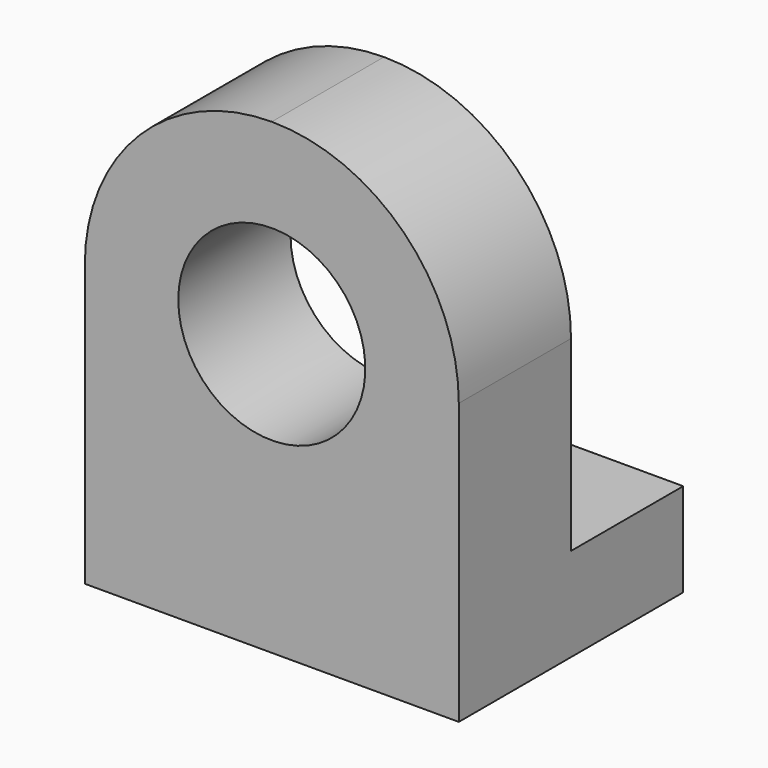
from build123d import *

# Parameters (mm, degrees)
F0_W     = 50.8
F0_H     = 38.1
F1_DEPTH = 6.35
F2_W     = 12.7
F2_H     = 12.7
F3_DEPTH = 12.701
F4_W     = 50.8
F4_H     = 19.05
F5_DEPTH = 50.8
F7_DEPTH = 19.051
F6_R     = 12.7
F8_DEPTH = 19.051


# Not quite as in the source:
# - a feature names something its author has since deleted; it is built from what else it names


with BuildPart() as f1:
    # F0 (on Top) → F1 (new body, symmetric)
    with BuildSketch(Plane.XY):
        Rectangle(F0_W, F0_H)
    extrude(amount=F1_DEPTH, both=True)

    # F2 (on face) → F3 (cut, through all)
    with BuildSketch(Plane.XY.offset(6.35)):
        with Locations((-19.05, 12.7)):
            Rectangle(F2_W, F2_H)
    extrude(amount=-F3_DEPTH, mode=Mode.SUBTRACT)

    # F4 (on face) → F5 (join)
    with BuildSketch(Plane.XY.offset(6.35)):
        with Locations((0, -9.525)):
            Rectangle(F4_W, F4_H)
    extrude(amount=F5_DEPTH)

    # F6 (on face) → F7 (cut, through all)
    with BuildSketch(Plane(origin=(0, 0, 0), x_dir=(-1, 0, 0), z_dir=(0, 1, 0))):
        with BuildLine():
            ThreePointArc((-25.4, 31.75), (-17.9605122618, 49.7105122225), (-5.57e-08, 57.15))
            Line((-5.57e-08, 57.15), (-25.4, 57.15))
            Line((-25.4, 57.15), (-25.4, 31.75))
        make_face()
        with BuildLine():
            ThreePointArc((-5.57e-08, 57.15), (17.9605122225, 49.7105122618), (25.4, 31.75))
            Line((25.4, 31.75), (25.4, 57.15))
            Line((25.4, 57.15), (-5.57e-08, 57.15))
        make_face()
    extrude(amount=-F7_DEPTH, mode=Mode.SUBTRACT)

    # F6 (on face) → F8 (cut, through all)
    with BuildSketch(Plane(origin=(0, 0, 0), x_dir=(-1, 0, 0), z_dir=(0, 1, 0))):
        with Locations((0, 31.75)):
            Circle(F6_R)
    extrude(amount=-F8_DEPTH, mode=Mode.SUBTRACT)


solid = f1.part
